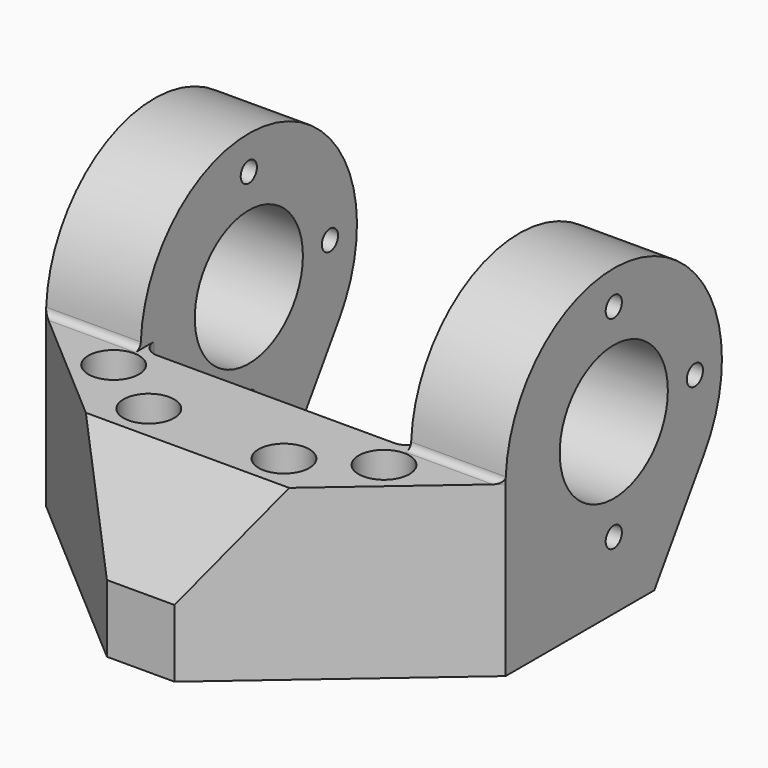
from build123d import *

# Parameters (mm, degrees)
F0_R        = 3
F0_R_2      = 20
F1_DEPTH    = 68
F2_W        = 40
F2_H        = 55
F3_DEPTH    = 90
F4_T4_DEPTH = 28
F4_T9_DEPTH = 28
F5_R        = 5
F6_R        = 7.5
F6_R_2      = 5
F7_DEPTH    = 10
F8_DEPTH    = 50


# Not quite as in the source:
# - a fillet or chamfer that OpenCascade refuses, or shapes differently, is made with other operations: its cross-section is extruded or revolved along the edge and cut away or added
# - a pattern or mirror of a feature is missing from the dataset's text; its kind, count and spacing are read off the source's solid


with BuildPart() as f1:
    # F0 (on Right) → F1 (new body, symmetric)
    with BuildSketch(Plane.YZ):
        with BuildLine():
            Line((-52.5, -26.7716136575), (52.5, -26.7716136575))
            Line((52.5, -26.7716136575), (70.9246015872, 1.2557668187))
            ThreePointArc((70.9246015872, 1.2557668187), (75.8209085454, 11.7606939741), (77.5, 23.2283863425))
            ThreePointArc((77.5, 23.2283863425), (37.5, 63.2283863425), (-2.5, 23.2283863425))
            Line((-2.5, 23.2283863425), (-35.1794919243, 23.2283863425))
            Line((-35.1794919243, 23.2283863425), (-52.5, -6.7716136575))
            Line((-52.5, -6.7716136575), (-52.5, -26.7716136575))
        make_face()
        with Locations((37.5, -6.7716136575)):
            Circle(F0_R, mode=Mode.SUBTRACT)
        with Locations((37.5, 23.2283863425)):
            Circle(F0_R_2, mode=Mode.SUBTRACT)
        with Locations((67.5, 23.2283863425)):
            Circle(F0_R, mode=Mode.SUBTRACT)
        with Locations((37.5, 53.2283863425)):
            Circle(F0_R, mode=Mode.SUBTRACT)
    extrude(amount=F1_DEPTH, both=True)

    # F2 (on face) → F3 (cut)
    with BuildSketch(Plane(origin=(0, 0, -26.7716136575), x_dir=(1, 0, 0), z_dir=(0, 0, -1))):
        Polygon((-40, -77.5), (40, -77.5), (40, 2.5), (0, 2.5), (0, -52.5), (-40, -52.5), align=None)
        with Locations((-20, -25)):
            Rectangle(F2_W, F2_H)
        Polygon((-68, 52.5), (-68, 2.5), (-10, 52.5), align=None)
    f3 = extrude(amount=-F3_DEPTH, mode=Mode.SUBTRACT)

    # F3_copies: F3 across plane
    add(f3.mirror(Plane(origin=(0, 0, 0), x_dir=(0, 0, 1), z_dir=(1, 0, 0))), mode=Mode.SUBTRACT)

    # F4: fillet of radius 2 on 2 edges, made by hand


with BuildPart() as f4_tool2:
    # F4_s3 → F4_t4 (new body)
    with BuildSketch(Plane.YZ.offset(-40)):
        with BuildLine():
            ThreePointArc((-4.4523539268, 23.2283863425), (-3.0722228081, 23.7808926136), (-2.4546227874, 25.1331482473))
            ThreePointArc((-2.4546227874, 25.1331482473), (-2.4886540877, 24.1810375123), (-2.5, 23.2283863425))
            Line((-2.5, 23.2283863425), (-4.4523539268, 23.2283863425))
        make_face()
    extrude(amount=-F4_T4_DEPTH)

    split(bisect_by=Plane(origin=(-30.2268076398, -35.0630968622, 0), x_dir=(0, 0, 1), z_dir=(0.6529396221, 0.7574099616, 0)), keep=Keep.TOP)


with BuildPart() as f1_1:
    add(f1.part)

    # F4_t1: union F4_tool2
    add(f4_tool2.part)


with BuildPart() as f4_tool7:
    # F4_s8 → F4_t9 (new body)
    with BuildSketch(Plane.YZ.offset(40)):
        with BuildLine():
            ThreePointArc((-4.4523539268, 23.2283863425), (-3.0722228081, 23.7808926136), (-2.4546227874, 25.1331482473))
            ThreePointArc((-2.4546227874, 25.1331482473), (-2.4886540877, 24.1810375123), (-2.5, 23.2283863425))
            Line((-2.5, 23.2283863425), (-4.4523539268, 23.2283863425))
        make_face()
    extrude(amount=F4_T9_DEPTH)

    split(bisect_by=Plane(origin=(30.2268076398, -35.0630968622, 0), x_dir=(0, 0, 1), z_dir=(-0.6529396221, 0.7574099616, 0)), keep=Keep.TOP)


with BuildPart() as f1_2:
    add(f1_1.part)

    # F4_t6: union F4_tool7
    add(f4_tool7.part)

    # F5
    f5_edges = [f1_2.edges().sort_by_distance(p)[0] for p in [
        (40, -2.5, -1.771614),
        (-40, -2.5, -1.771614),
    ]]
    fillet(f5_edges, radius=F5_R)

    # F6 (on face) → F7 (cut)
    with BuildSketch(Plane.XY.offset(23.2283863425)):
        with Locations((40, -12.5)):
            Circle(F6_R)
        with Locations((40, -12.5)):
            Circle(F6_R_2, mode=Mode.SUBTRACT)
        with Locations((20, -24.5)):
            Circle(F6_R)
        with Locations((20, -24.5)):
            Circle(F6_R_2, mode=Mode.SUBTRACT)
        with Locations((-20, -24.5)):
            Circle(F6_R)
        with Locations((-20, -24.5)):
            Circle(F6_R_2, mode=Mode.SUBTRACT)
        with Locations((-40, -12.5)):
            Circle(F6_R)
        with Locations((-40, -12.5)):
            Circle(F6_R_2, mode=Mode.SUBTRACT)
    extrude(amount=-F7_DEPTH, mode=Mode.SUBTRACT)

    # F8 (cut): faces of the model
    f8_faces = [f1_2.faces().sort_by_distance(p)[0] for p in [
        (-40, -12.5, 23.2283863425),
        (-20, -24.5, 23.2283863425),
        (20, -24.5, 23.2283863425),
        (40, -12.5, 23.2283863425),
    ]]
    extrude(f8_faces, amount=-F8_DEPTH, mode=Mode.SUBTRACT)


solid = f1_2.part
